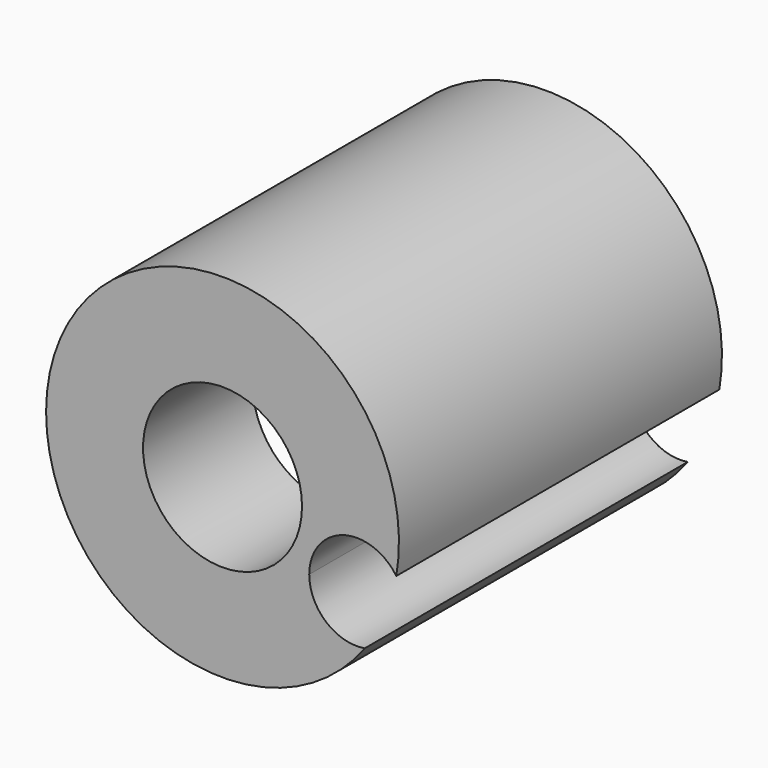
from build123d import *

# Parameters (mm, degrees)
F0_R     = 11.1
F0_R_2   = 5
F1_DEPTH = 25.4
F2_W     = 16.7754087597
F2_H     = 27.2372085601
F3_DEPTH = 76.2
F5_DEPTH = 25.401


with BuildPart() as f1:
    # F0 (on Front) → F1 (new body)
    with BuildSketch(Plane.XZ):
        Circle(F0_R)
        Circle(F0_R_2, mode=Mode.SUBTRACT)
    extrude(amount=F1_DEPTH)

    # F2 (on Right) → F3 (cut)
    with BuildSketch(Plane.YZ):
        with Locations((-8.3877043799, -13.6186042801)):
            Rectangle(F2_W, F2_H)
    extrude(amount=-F3_DEPTH, mode=Mode.SUBTRACT)

    # F4 (on face) → F5 (cut, through all)
    with BuildSketch(Plane(origin=(0, 0, 0), x_dir=(-1, 0, 0), z_dir=(0, 1, 0))):
        with BuildLine():
            ThreePointArc((-8.9445990977, -6.572986154), (-6.5138225835, -5.901619973), (-5.4539214149, -3.6133856047))
            ThreePointArc((-5.4539214149, -3.6133856047), (-7.5692818154, -0.7467826013), (-10.9321966009, -1.9227785828))
            ThreePointArc((-10.9321966009, -1.9227785828), (-10.2067555778, -4.3625841625), (-8.9445990977, -6.572986154))
        make_face()
    extrude(amount=-F5_DEPTH, mode=Mode.SUBTRACT)


solid = f1.part
